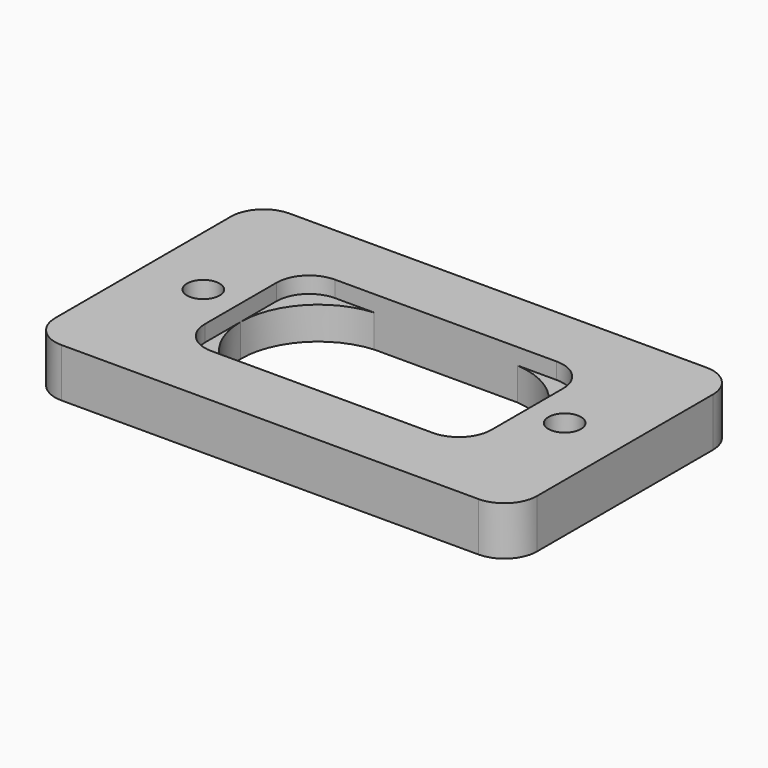
from build123d import *

# Parameters (mm, degrees)
F1_DEPTH = 3
F2_DEPTH = 2
F3_R     = 2
F6_D     = 2


# Not quite as in the source:
# - a feature names something its author has since deleted; it is built from what else it names


with BuildPart() as f1:
    # F0 (on Top) → F1 (new body)
    with BuildSketch(Plane.XY):
        Polygon((-4.4, 4.75), (0, 4.75), (0, 8.75), (-14.8, 8.75), (-14.8, 0), (-8.8, 0), (-8.8, 4.75), align=None)
    extrude(amount=F1_DEPTH)

    # F0 (on Top) → F2 (join)
    with BuildSketch(Plane.XY):
        with BuildLine():
            ThreePointArc((-8.8, 0), (-7.5309776981, 3.2373793414), (-4.4, 4.75))
            Line((-4.4, 4.75), (-8.8, 4.75))
            Line((-8.8, 4.75), (-8.8, 0))
        make_face()
    extrude(amount=F2_DEPTH)

    # F3
    f3_edges = [f1.edges().sort_by_distance(p)[0] for p in [
        (-14.8, 8.75, 1.5),
        (-8.8, 4.75, 2.5),
    ]]
    fillet(f3_edges, radius=F3_R)

    # F4: F1 across face


with BuildPart() as f1_1:
    add(f1.part)
    add(f1.part.mirror(Plane(origin=(-11.8, 0, 1.5), x_dir=(1, 0, 0), z_dir=(0, -1, 0))))

    # F6 (through all)
    with Locations(Plane.XY.offset(3)):
        with Locations((-11.1, 0)):
            Hole(F6_D / 2)

    # F7: F1 across face


with BuildPart() as f1_2:
    add(f1_1.part)
    add(f1_1.part.mirror(Plane(origin=(0, 6.75, 1.5), x_dir=(0, 1, 0), z_dir=(1, 0, 0))))


solid = f1_2.part
